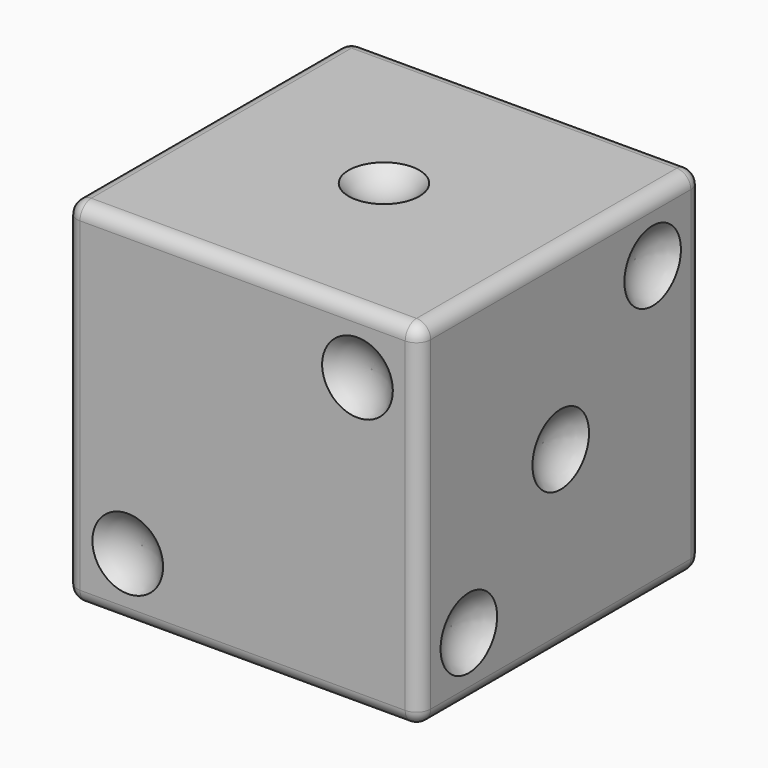
from build123d import *

# Parameters (mm, degrees)
F0_W      = 127
F0_H      = 127
F1_DEPTH  = 127
F2_R      = 12.7
F3_DEPTH  = 6.35
F4_R      = 12.7
F5_DEPTH  = 6.35
F6_R      = 12.7
F7_DEPTH  = 6.35
F8_R      = 12.7
F9_DEPTH  = 6.35
F11_R     = 12.7
F12_DEPTH = 6.35
F10_R     = 12.7
F13_DEPTH = 6.35
F14_R     = 5.08


# Not quite as in the source:
# - a fillet or chamfer that OpenCascade refuses, or shapes differently, is made with other operations: its cross-section is extruded or revolved along the edge and cut away or added


with BuildPart() as f1:
    # F0 (on Front) → F1 (new body)
    with BuildSketch(Plane.XZ):
        with Locations((63.5, 63.5)):
            Rectangle(F0_W, F0_H)
    extrude(amount=F1_DEPTH)

    # F2 (on face) → F3 (cut)
    with BuildSketch(Plane.XY.offset(127)):
        with Locations((63.5, -63.5)):
            Circle(F2_R)
    extrude(amount=-F3_DEPTH, mode=Mode.SUBTRACT)

    # F4 (on face) → F5 (cut)
    with BuildSketch(Plane.XZ.offset(127)):
        with Locations((22.225, 22.225)):
            Circle(F4_R)
        with Locations((104.775, 104.775)):
            Circle(F4_R)
    extrude(amount=-F5_DEPTH, mode=Mode.SUBTRACT)

    # F6 (on face) → F7 (cut)
    with BuildSketch(Plane(origin=(0, 0, 0), x_dir=(1, 0, 0), z_dir=(0, 0, -1))):
        with Locations((104.775, 104.775)):
            Circle(F6_R)
        with Locations((104.775, 22.225)):
            Circle(F6_R)
        with Locations((22.225, 104.775)):
            Circle(F6_R)
        with Locations((22.225, 22.225)):
            Circle(F6_R)
        with Locations((63.5, 104.775)):
            Circle(F6_R)
        with Locations((63.5, 22.225)):
            Circle(F6_R)
    extrude(amount=-F7_DEPTH, mode=Mode.SUBTRACT)

    # F8 (on face) → F9 (cut)
    with BuildSketch(Plane(origin=(0, 0, 0), x_dir=(-1, 0, 0), z_dir=(0, 1, 0))):
        with Locations((-104.775, 104.775)):
            Circle(F8_R)
        with Locations((-22.225, 104.775)):
            Circle(F8_R)
        with Locations((-104.775, 22.225)):
            Circle(F8_R)
        with Locations((-22.225, 22.225)):
            Circle(F8_R)
        with Locations((-63.5, 63.5)):
            Circle(F8_R)
    extrude(amount=-F9_DEPTH, mode=Mode.SUBTRACT)

    # F11 (on face) → F12 (cut)
    with BuildSketch(Plane.YZ.offset(127)):
        with Locations((-22.225, 104.775)):
            Circle(F11_R)
        with Locations((-104.775, 22.225)):
            Circle(F11_R)
        with Locations((-63.5, 63.5)):
            Circle(F11_R)
    extrude(amount=-F12_DEPTH, mode=Mode.SUBTRACT)

    # F10 (on face) → F13 (cut)
    with BuildSketch(Plane(origin=(0, 0, 0), x_dir=(0, -1, 0), z_dir=(-1, 0, 0))):
        with Locations((22.225, 22.225)):
            Circle(F10_R)
        with Locations((22.225, 104.775)):
            Circle(F10_R)
        with Locations((104.775, 22.225)):
            Circle(F10_R)
        with Locations((104.775, 104.775)):
            Circle(F10_R)
    extrude(amount=-F13_DEPTH, mode=Mode.SUBTRACT)

    # F14
    f14_edges = [f1.edges().sort_by_distance(p)[0] for p in [
        (127, -127, 63.5),
        (127, -63.5, 127),
        (63.5, -127, 127),
        (0, -127, 63.5),
        (0, -63.5, 127),
        (63.5, -127, 0),
        (0, -63.5, 0),
        (63.5, 0, 0),
        (0, 0, 63.5),
        (127, -63.5, 0),
        (63.5, 0, 127),
        (127, 0, 63.5),
    ]]
    fillet(f14_edges, radius=F14_R)

    # F15: fillet of radius 15.494 on 21 edges, made by hand

    # F15_s1 → F15_t2 (revolve)
    with BuildSketch(Plane.XY.offset(104.775)):
        with BuildLine():
            ThreePointArc((117.475, -127), (111.9807548376, -122.3284078665), (104.9669505917, -120.65))
            Line((104.9669505917, -120.65), (117.475, -120.65))
            Line((117.475, -120.65), (117.475, -127))
        make_face()
    revolve(axis=Axis((104.775, -120.65, 104.775), (0, -1, 0)))

    # F15_s3 → F15_t4 (revolve)
    with BuildSketch(Plane.XY.offset(22.225)):
        with BuildLine():
            ThreePointArc((34.925, -127), (29.4307548376, -122.3284078665), (22.4169505917, -120.65))
            Line((22.4169505917, -120.65), (34.925, -120.65))
            Line((34.925, -120.65), (34.925, -127))
        make_face()
    revolve(axis=Axis((22.225, -120.65, 22.225), (0, -1, 0)))

    # F15_s5 → F15_t6 (revolve)
    with BuildSketch(Plane.XY.offset(22.225)):
        with BuildLine():
            ThreePointArc((127, -92.075), (122.3284078665, -97.5692451624), (120.65, -104.5830494083))
            Line((120.65, -104.5830494083), (120.65, -92.075))
            Line((120.65, -92.075), (127, -92.075))
        make_face()
    revolve(axis=Axis((120.65, -104.775, 22.225), (1, 0, 0)))

    # F15_s7 → F15_t8 (revolve)
    with BuildSketch(Plane.XY.offset(63.5)):
        with BuildLine():
            ThreePointArc((127, -50.8), (122.3284078665, -56.2942451624), (120.65, -63.3080494083))
            Line((120.65, -63.3080494083), (120.65, -50.8))
            Line((120.65, -50.8), (127, -50.8))
        make_face()
    revolve(axis=Axis((120.65, -63.5, 63.5), (1, 0, 0)))

    # F15_s9 → F15_t10 (revolve)
    with BuildSketch(Plane.XY.offset(104.775)):
        with BuildLine():
            ThreePointArc((127, -9.525), (122.3284078665, -15.0192451624), (120.65, -22.0330494083))
            Line((120.65, -22.0330494083), (120.65, -9.525))
            Line((120.65, -9.525), (127, -9.525))
        make_face()
    revolve(axis=Axis((120.65, -22.225, 104.775), (1, 0, 0)))

    # F15_s11 → F15_t12 (revolve)
    with BuildSketch(Plane.XZ.offset(63.5)):
        with BuildLine():
            ThreePointArc((76.2, 127), (70.7057548376, 122.3284078665), (63.6919505917, 120.65))
            Line((63.6919505917, 120.65), (76.2, 120.65))
            Line((76.2, 120.65), (76.2, 127))
        make_face()
    revolve(axis=Axis((63.5, -63.5, 120.65), (0, 0, 1)))

    # F15_s13 → F15_t14 (revolve)
    with BuildSketch(Plane.XY.offset(104.775)):
        with BuildLine():
            ThreePointArc((92.075, 0), (97.5692451624, -4.6715921335), (104.5830494083, -6.35))
            Line((104.5830494083, -6.35), (92.075, -6.35))
            Line((92.075, -6.35), (92.075, 0))
        make_face()
    revolve(axis=Axis((104.775, -6.35, 104.775), (0, 1, 0)))

    # F15_s15 → F15_t16 (revolve)
    with BuildSketch(Plane.XY.offset(104.775)):
        with BuildLine():
            ThreePointArc((9.525, 0), (15.0192451624, -4.6715921335), (22.0330494083, -6.35))
            Line((22.0330494083, -6.35), (9.525, -6.35))
            Line((9.525, -6.35), (9.525, 0))
        make_face()
    revolve(axis=Axis((22.225, -6.35, 104.775), (0, 1, 0)))

    # F15_s17 → F15_t18 (revolve)
    with BuildSketch(Plane.XY.offset(63.5)):
        with BuildLine():
            ThreePointArc((50.8, 0), (56.2942451624, -4.6715921335), (63.3080494083, -6.35))
            Line((63.3080494083, -6.35), (50.8, -6.35))
            Line((50.8, -6.35), (50.8, 0))
        make_face()
    revolve(axis=Axis((63.5, -6.35, 63.5), (0, 1, 0)))

    # F15_s19 → F15_t20 (revolve)
    with BuildSketch(Plane.XY.offset(22.225)):
        with BuildLine():
            ThreePointArc((92.075, 0), (97.5692451624, -4.6715921335), (104.5830494083, -6.35))
            Line((104.5830494083, -6.35), (92.075, -6.35))
            Line((92.075, -6.35), (92.075, 0))
        make_face()
    revolve(axis=Axis((104.775, -6.35, 22.225), (0, 1, 0)))

    # F15_s21 → F15_t22 (revolve)
    with BuildSketch(Plane.XY.offset(22.225)):
        with BuildLine():
            ThreePointArc((9.525, 0), (15.0192451624, -4.6715921335), (22.0330494083, -6.35))
            Line((22.0330494083, -6.35), (9.525, -6.35))
            Line((9.525, -6.35), (9.525, 0))
        make_face()
    revolve(axis=Axis((22.225, -6.35, 22.225), (0, 1, 0)))

    # F15_s23 → F15_t24 (revolve)
    with BuildSketch(Plane.XY.offset(104.775)):
        with BuildLine():
            ThreePointArc((0, -34.925), (4.6715921335, -29.4307548376), (6.35, -22.4169505917))
            Line((6.35, -22.4169505917), (6.35, -34.925))
            Line((6.35, -34.925), (0, -34.925))
        make_face()
    revolve(axis=Axis((6.35, -22.225, 104.775), (-1, 0, 0)))

    # F15_s25 → F15_t26 (revolve)
    with BuildSketch(Plane.XY.offset(104.775)):
        with BuildLine():
            ThreePointArc((0, -117.475), (4.6715921335, -111.9807548376), (6.35, -104.9669505917))
            Line((6.35, -104.9669505917), (6.35, -117.475))
            Line((6.35, -117.475), (0, -117.475))
        make_face()
    revolve(axis=Axis((6.35, -104.775, 104.775), (-1, 0, 0)))

    # F15_s27 → F15_t28 (revolve)
    with BuildSketch(Plane.XY.offset(22.225)):
        with BuildLine():
            ThreePointArc((0, -117.475), (4.6715921335, -111.9807548376), (6.35, -104.9669505917))
            Line((6.35, -104.9669505917), (6.35, -117.475))
            Line((6.35, -117.475), (0, -117.475))
        make_face()
    revolve(axis=Axis((6.35, -104.775, 22.225), (-1, 0, 0)))

    # F15_s29 → F15_t30 (revolve)
    with BuildSketch(Plane.XY.offset(22.225)):
        with BuildLine():
            ThreePointArc((0, -34.925), (4.6715921335, -29.4307548376), (6.35, -22.4169505917))
            Line((6.35, -22.4169505917), (6.35, -34.925))
            Line((6.35, -34.925), (0, -34.925))
        make_face()
    revolve(axis=Axis((6.35, -22.225, 22.225), (-1, 0, 0)))

    # F15_s31 → F15_t32 (revolve)
    with BuildSketch(Plane.XZ.offset(104.775)):
        with BuildLine():
            ThreePointArc((34.925, 0), (29.4307548376, 4.6715921335), (22.4169505917, 6.35))
            Line((22.4169505917, 6.35), (34.925, 6.35))
            Line((34.925, 6.35), (34.925, 0))
        make_face()
    revolve(axis=Axis((22.225, -104.775, 6.35), (0, 0, -1)))

    # F15_s33 → F15_t34 (revolve)
    with BuildSketch(Plane.XZ.offset(104.775)):
        with BuildLine():
            ThreePointArc((76.2, 0), (70.7057548376, 4.6715921335), (63.6919505917, 6.35))
            Line((63.6919505917, 6.35), (76.2, 6.35))
            Line((76.2, 6.35), (76.2, 0))
        make_face()
    revolve(axis=Axis((63.5, -104.775, 6.35), (0, 0, -1)))

    # F15_s35 → F15_t36 (revolve)
    with BuildSketch(Plane.XZ.offset(104.775)):
        with BuildLine():
            ThreePointArc((117.475, 0), (111.9807548376, 4.6715921335), (104.9669505917, 6.35))
            Line((104.9669505917, 6.35), (117.475, 6.35))
            Line((117.475, 6.35), (117.475, 0))
        make_face()
    revolve(axis=Axis((104.775, -104.775, 6.35), (0, 0, -1)))

    # F15_s37 → F15_t38 (revolve)
    with BuildSketch(Plane.XZ.offset(22.225)):
        with BuildLine():
            ThreePointArc((117.475, 0), (111.9807548376, 4.6715921335), (104.9669505917, 6.35))
            Line((104.9669505917, 6.35), (117.475, 6.35))
            Line((117.475, 6.35), (117.475, 0))
        make_face()
    revolve(axis=Axis((104.775, -22.225, 6.35), (0, 0, -1)))

    # F15_s39 → F15_t40 (revolve)
    with BuildSketch(Plane.XZ.offset(22.225)):
        with BuildLine():
            ThreePointArc((76.2, 0), (70.7057548376, 4.6715921335), (63.6919505917, 6.35))
            Line((63.6919505917, 6.35), (76.2, 6.35))
            Line((76.2, 6.35), (76.2, 0))
        make_face()
    revolve(axis=Axis((63.5, -22.225, 6.35), (0, 0, -1)))

    # F15_s41 → F15_t42 (revolve)
    with BuildSketch(Plane.XZ.offset(22.225)):
        with BuildLine():
            ThreePointArc((34.925, 0), (29.4307548376, 4.6715921335), (22.4169505917, 6.35))
            Line((22.4169505917, 6.35), (34.925, 6.35))
            Line((34.925, 6.35), (34.925, 0))
        make_face()
    revolve(axis=Axis((22.225, -22.225, 6.35), (0, 0, -1)))


solid = f1.part
